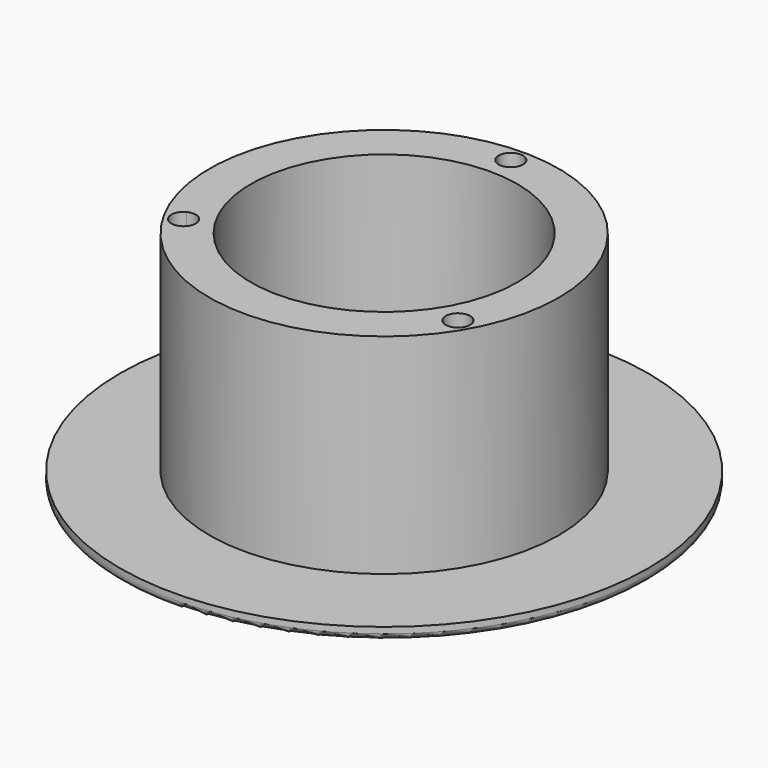
from build123d import *

# Parameters (mm, degrees)
F0_R     = 21.5
F0_R_2   = 16.4
F1_DEPTH = 27.25
F0_R_3   = 32.5
F2_DEPTH = 1.5
F0_R_4   = 14.2
F3_DEPTH = 1
F5_DEPTH = 5
F6_R     = 0.75
F7_SIZE  = 0.99999
F8_DEPTH = 1


# Not quite as in the source:
# - a fillet or chamfer is up to 0.001 mm smaller than in the source, because OpenCascade refuses the exact size


with BuildPart() as f1:
    # F0 (on Top) → F1 (new body)
    with BuildSketch(Plane.XY):
        Circle(F0_R)
        Circle(F0_R_2, mode=Mode.SUBTRACT)
    extrude(amount=F1_DEPTH)

    # F0 (on Top) → F2 (join)
    with BuildSketch(Plane.XY):
        Circle(F0_R_3)
        Circle(F0_R, mode=Mode.SUBTRACT)
    extrude(amount=F2_DEPTH)

    # F0 (on Top) → F3 (join)
    with BuildSketch(Plane.XY):
        Circle(F0_R_2)
        Circle(F0_R_4, mode=Mode.SUBTRACT)
    extrude(amount=F3_DEPTH)

    # F4 (on face) → F5 (cut)
    with BuildSketch(Plane.XY.offset(27.25)):
        with BuildLine():
            ThreePointArc((-1.4988901219, 19.4423076923), (0, 18), (1.4988901219, 19.4423076923))
            ThreePointArc((1.4988901219, 19.4423076923), (0, 19.5), (-1.4988901219, 19.4423076923))
        make_face()
        with BuildLine():
            ThreePointArc((-1.4988901219, 19.4423076923), (0, 19.5), (1.4988901219, 19.4423076923))
            ThreePointArc((1.4988901219, 19.4423076923), (1.4997225048, 19.4711485087), (1.5, 19.5))
            ThreePointArc((1.5, 19.5), (-0.0288514913, 20.9997225048), (-1.4988901219, 19.4423076923))
        make_face()
        with BuildLine():
            ThreePointArc((18.3874953738, -9.75), (18.171867416, -8.9751526232), (17.5869774307, -8.4230769231))
            ThreePointArc((17.5869774307, -8.4230769231), (16.8874953738, -9.75), (16.0880873088, -11.0192307692))
            ThreePointArc((16.0880873088, -11.0192307692), (17.6123705018, -11.0632235334), (18.3874953738, -9.75))
        make_face()
        with BuildLine():
            ThreePointArc((16.0880873088, -11.0192307692), (16.8874953738, -9.75), (17.5869774307, -8.4230769231))
            ThreePointArc((17.5869774307, -8.4230769231), (15.5884572681, -9), (16.0880873088, -11.0192307692))
        make_face()
        with BuildLine():
            ThreePointArc((-15.3874953738, -9.75), (-16.112647997, -8.4656279578), (-17.5869774307, -8.4230769231))
            ThreePointArc((-17.5869774307, -8.4230769231), (-16.8874953738, -9.75), (-16.0880873088, -11.0192307692))
            ThreePointArc((-16.0880873088, -11.0192307692), (-15.5742718404, -10.474875128), (-15.3874953738, -9.75))
        make_face()
        with BuildLine():
            ThreePointArc((-16.0880873088, -11.0192307692), (-16.8874953738, -9.75), (-17.5869774307, -8.4230769231))
            ThreePointArc((-17.5869774307, -8.4230769231), (-18.1865334795, -10.5), (-16.0880873088, -11.0192307692))
        make_face()
    extrude(amount=-F5_DEPTH, mode=Mode.SUBTRACT)

    # F6
    f6_edges = [f1.edges().sort_by_distance(p)[0] for p in [
        (-32.5, 0, 0),
    ]]
    fillet(f6_edges, radius=F6_R)

    # F7 (size 1 in the source; OpenCascade refuses exactly that, so slightly less here)
    f7_edges = [f1.edges().sort_by_distance(p)[0] for p in [
        (-14.2, 0, 0),
    ]]
    chamfer(f7_edges, length=F7_SIZE)

    # F8 (add): a face of the model
    f8_faces = [f1.faces().sort_by_distance(p)[0] for p in [
        (-15.9361379515, 0, 1),
    ]]
    extrude(f8_faces, amount=F8_DEPTH)


solid = f1.part
